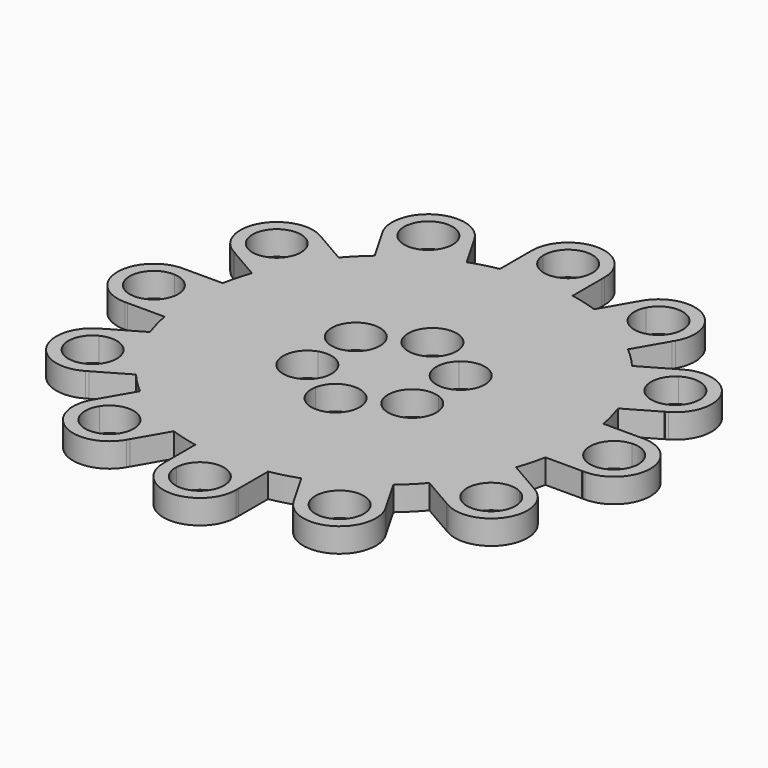
from build123d import *

# Parameters (mm, degrees)
F1_DEPTH = 1


with BuildPart() as f1:
    # F0 (on Top) → F1 (new body)
    with BuildSketch(Plane.XY):
        with BuildLine():
            ThreePointArc((9.4473684211, -0.9986139979), (8.5, 0), (9.4473684211, 0.9986139979))
            ThreePointArc((9.4473684211, 0.9986139979), (9.4177488558, 1.2473998912), (9.3815789474, 1.4953181783))
            ThreePointArc((9.3815789474, 1.4953181783), (9.3812055256, 1.4976591358), (9.3808315196, 1.5))
            Line((9.3808315196, 1.5), (7.8581168228, 1.5))
            ThreePointArc((7.8581168228, 1.5), (7.964450219, 0.7533476681), (8, 0))
            ThreePointArc((8, 0), (7.964450219, -0.7533476681), (7.8581168228, -1.5))
            Line((7.8581168228, -1.5), (9.3808315196, -1.5))
            ThreePointArc((9.3808315196, -1.5), (9.3812055256, -1.4976591358), (9.3815789474, -1.4953181783))
            ThreePointArc((9.3815789474, -1.4953181783), (9.4177488558, -1.2473998912), (9.4473684211, -0.9986139979))
        make_face()
        with BuildLine():
            ThreePointArc((9.3815789474, 1.4953181783), (9.4177488558, 1.2473998912), (9.4473684211, 0.9986139979))
            ThreePointArc((9.4473684211, 0.9986139979), (10.1882472016, 0.7254762501), (10.5, 0))
            ThreePointArc((10.5, 0), (10.1882472016, -0.7254762501), (9.4473684211, -0.9986139979))
            ThreePointArc((9.4473684211, -0.9986139979), (9.4177488558, -1.2473998912), (9.3815789474, -1.4953181783))
            ThreePointArc((9.3815789474, -1.4953181783), (9.4407432173, -1.4988290876), (9.5, -1.5))
            ThreePointArc((9.5, -1.5), (11, 0), (9.5, 1.5))
            ThreePointArc((9.5, 1.5), (9.4407432173, 1.4988290876), (9.3815789474, 1.4953181783))
        make_face()
        with BuildLine():
            Line((7.5553287944, 2.6300203057), (8.8740384046, 3.3913776541))
            ThreePointArc((8.8740384046, 3.3913776541), (8.8731918712, 3.393591905), (8.8723447852, 3.3958059446))
            ThreePointArc((8.8723447852, 3.3958059446), (8.7797097012, 3.6285944334), (8.6809680505, 3.8588591197))
            ThreePointArc((8.6809680505, 3.8588591197), (7.3612159322, 4.25), (7.6823540526, 5.5885093013))
            ThreePointArc((7.6823540526, 5.5885093013), (7.53230981, 5.7891544224), (7.3770266069, 5.9857730028))
            ThreePointArc((7.3770266069, 5.9857730028), (7.3755327354, 5.9876136206), (7.3740384046, 5.9894538655))
            Line((7.3740384046, 5.9894538655), (6.0553287944, 5.2280965171))
            ThreePointArc((6.0553287944, 5.2280965171), (6.9282032303, 4), (7.5553287944, 2.6300203057))
        make_face()
        with BuildLine():
            ThreePointArc((8, 0), (7.964450219, 0.7533476681), (7.8581168228, 1.5))
            ThreePointArc((7.8581168228, 1.5), (7.7274066103, 2.0705523608), (7.5553287944, 2.6300203057))
            ThreePointArc((7.5553287944, 2.6300203057), (6.9282032303, 4), (6.0553287944, 5.2280965171))
            ThreePointArc((6.0553287944, 5.2280965171), (5.6568542495, 5.6568542495), (5.2280965171, 6.0553287944))
            ThreePointArc((5.2280965171, 6.0553287944), (4, 6.9282032303), (2.6300203057, 7.5553287944))
            ThreePointArc((2.6300203057, 7.5553287944), (2.0705523608, 7.7274066103), (1.5, 7.8581168228))
            ThreePointArc((1.5, 7.8581168228), (0, 8), (-1.5, 7.8581168228))
            ThreePointArc((-1.5, 7.8581168228), (-2.0705523608, 7.7274066103), (-2.6300203057, 7.5553287944))
            ThreePointArc((-2.6300203057, 7.5553287944), (-4, 6.9282032303), (-5.2280965171, 6.0553287944))
            ThreePointArc((-5.2280965171, 6.0553287944), (-5.6568542495, 5.6568542495), (-6.0553287944, 5.2280965171))
            ThreePointArc((-6.0553287944, 5.2280965171), (-6.9282032303, 4), (-7.5553287944, 2.6300203057))
            ThreePointArc((-7.5553287944, 2.6300203057), (-7.7274066103, 2.0705523608), (-7.8581168228, 1.5))
            ThreePointArc((-7.8581168228, 1.5), (-8, 0), (-7.8581168228, -1.5))
            ThreePointArc((-7.8581168228, -1.5), (-7.7274066103, -2.0705523608), (-7.5553287944, -2.6300203057))
            ThreePointArc((-7.5553287944, -2.6300203057), (-6.9282032303, -4), (-6.0553287944, -5.2280965171))
            ThreePointArc((-6.0553287944, -5.2280965171), (-5.6568542495, -5.6568542495), (-5.2280965171, -6.0553287944))
            ThreePointArc((-5.2280965171, -6.0553287944), (-4, -6.9282032303), (-2.6300203057, -7.5553287944))
            ThreePointArc((-2.6300203057, -7.5553287944), (-2.0705523608, -7.7274066103), (-1.5, -7.8581168228))
            ThreePointArc((-1.5, -7.8581168228), (0, -8), (1.5, -7.8581168228))
            ThreePointArc((1.5, -7.8581168228), (2.0705523608, -7.7274066103), (2.6300203057, -7.5553287944))
            ThreePointArc((2.6300203057, -7.5553287944), (4, -6.9282032303), (5.2280965171, -6.0553287944))
            ThreePointArc((5.2280965171, -6.0553287944), (5.6568542495, -5.6568542495), (6.0553287944, -5.2280965171))
            ThreePointArc((6.0553287944, -5.2280965171), (6.9282032303, -4), (7.5553287944, -2.6300203057))
            ThreePointArc((7.5553287944, -2.6300203057), (7.7274066103, -2.0705523608), (7.8581168228, -1.5))
            ThreePointArc((7.8581168228, -1.5), (7.964450219, -0.7533476681), (8, 0))
        make_face()
        with BuildLine():
            ThreePointArc((2.4817563773, 0.3014718626), (2.4954349263, 0.1510116831), (2.5, 0))
            ThreePointArc((2.5, 0), (2.4954349263, -0.1510116831), (2.4817563773, -0.3014718626))
            ThreePointArc((2.4817563773, -0.3014718626), (2.9764490121, -0.6654886091), (3.1650635095, -1.25))
            ThreePointArc((3.1650635095, -1.25), (2.5754882716, -2.1618944646), (1.5019604801, -1.9985281374))
            ThreePointArc((1.5019604801, -1.9985281374), (1.25, -2.1650635095), (0.9797958971, -2.3))
            ThreePointArc((0.9797958971, -2.3), (0.994936153, -2.399491038), (1, -2.5))
            ThreePointArc((1, -2.5), (-0.100508962, -3.494936153), (-0.9797958971, -2.3))
            ThreePointArc((-0.9797958971, -2.3), (-1.25, -2.1650635095), (-1.5019604801, -1.9985281374))
            ThreePointArc((-1.5019604801, -1.9985281374), (-3.0310889132, -1.75), (-2.4817563773, -0.3014718626))
            ThreePointArc((-2.4817563773, -0.3014718626), (-2.5, 0), (-2.4817563773, 0.3014718626))
            ThreePointArc((-2.4817563773, 0.3014718626), (-3.0310889132, 1.75), (-1.5019604801, 1.9985281374))
            ThreePointArc((-1.5019604801, 1.9985281374), (-1.25, 2.1650635095), (-0.9797958971, 2.3))
            ThreePointArc((-0.9797958971, 2.3), (-0.100508962, 3.494936153), (1, 2.5))
            ThreePointArc((1, 2.5), (0.994936153, 2.399491038), (0.9797958971, 2.3))
            ThreePointArc((0.9797958971, 2.3), (1.25, 2.1650635095), (1.5019604801, 1.9985281374))
            ThreePointArc((1.5019604801, 1.9985281374), (2.5754882716, 2.1618944646), (3.1650635095, 1.25))
            ThreePointArc((3.1650635095, 1.25), (2.9764490121, 0.6654886091), (2.4817563773, 0.3014718626))
        make_face(mode=Mode.SUBTRACT)
        with BuildLine():
            ThreePointArc((8.8723447852, -3.3958059446), (8.8731918712, -3.393591905), (8.8740384046, -3.3913776541))
            Line((8.8740384046, -3.3913776541), (7.5553287944, -2.6300203057))
            ThreePointArc((7.5553287944, -2.6300203057), (6.9282032303, -4), (6.0553287944, -5.2280965171))
            Line((6.0553287944, -5.2280965171), (7.3740384046, -5.9894538655))
            ThreePointArc((7.3740384046, -5.9894538655), (7.3755327354, -5.9876136206), (7.3770266069, -5.9857730028))
            ThreePointArc((7.3770266069, -5.9857730028), (7.53230981, -5.7891544224), (7.6823540526, -5.5885093013))
            ThreePointArc((7.6823540526, -5.5885093013), (7.3612159322, -4.25), (8.6809680505, -3.8588591197))
            ThreePointArc((8.6809680505, -3.8588591197), (8.7797097012, -3.6285944334), (8.8723447852, -3.3958059446))
        make_face()
        with BuildLine():
            ThreePointArc((8.6809680505, 3.8588591197), (8.7797097012, 3.6285944334), (8.8723447852, 3.3958059446))
            ThreePointArc((8.8723447852, 3.3958059446), (8.9253380006, 3.4223475429), (8.977241336, 3.4509618943))
            ThreePointArc((8.977241336, 3.4509618943), (9.5262794416, 5.5), (7.477241336, 6.0490381057))
            ThreePointArc((7.477241336, 6.0490381057), (7.4265089131, 6.0183956744), (7.3770266069, 5.9857730028))
            ThreePointArc((7.3770266069, 5.9857730028), (7.53230981, 5.7891544224), (7.6823540526, 5.5885093013))
            ThreePointArc((7.6823540526, 5.5885093013), (8.7042700126, 5.6288877299), (9.227241336, 4.75))
            ThreePointArc((9.227241336, 4.75), (9.0798041532, 4.2273752372), (8.6809680505, 3.8588591197))
        make_face()
        with BuildLine():
            ThreePointArc((8.977241336, -3.4509618943), (8.9253380006, -3.4223475429), (8.8723447852, -3.3958059446))
            ThreePointArc((8.8723447852, -3.3958059446), (8.7797097012, -3.6285944334), (8.6809680505, -3.8588591197))
            ThreePointArc((8.6809680505, -3.8588591197), (9.0798041532, -4.2273752372), (9.227241336, -4.75))
            ThreePointArc((9.227241336, -4.75), (8.7042700126, -5.6288877299), (7.6823540526, -5.5885093013))
            ThreePointArc((7.6823540526, -5.5885093013), (7.53230981, -5.7891544224), (7.3770266069, -5.9857730028))
            ThreePointArc((7.3770266069, -5.9857730028), (7.4265089131, -6.0183956744), (7.477241336, -6.0490381057))
            ThreePointArc((7.477241336, -6.0490381057), (9.5262794416, -5.5), (8.977241336, -3.4509618943))
        make_face()
        with BuildLine():
            ThreePointArc((2.6300203057, 7.5553287944), (4, 6.9282032303), (5.2280965171, 6.0553287944))
            Line((5.2280965171, 6.0553287944), (5.9894538655, 7.3740384046))
            ThreePointArc((5.9894538655, 7.3740384046), (5.9876136206, 7.3755327354), (5.9857730028, 7.3770266069))
            ThreePointArc((5.9857730028, 7.3770266069), (5.7891544224, 7.53230981), (5.5885093013, 7.6823540526))
            ThreePointArc((5.5885093013, 7.6823540526), (4.25, 7.3612159322), (3.8588591197, 8.6809680505))
            ThreePointArc((3.8588591197, 8.6809680505), (3.6285944334, 8.7797097012), (3.3958059446, 8.8723447852))
            ThreePointArc((3.3958059446, 8.8723447852), (3.393591905, 8.8731918712), (3.3913776541, 8.8740384046))
            Line((3.3913776541, 8.8740384046), (2.6300203057, 7.5553287944))
        make_face()
        with BuildLine():
            Line((5.9894538655, -7.3740384046), (5.2280965171, -6.0553287944))
            ThreePointArc((5.2280965171, -6.0553287944), (4, -6.9282032303), (2.6300203057, -7.5553287944))
            Line((2.6300203057, -7.5553287944), (3.3913776541, -8.8740384046))
            ThreePointArc((3.3913776541, -8.8740384046), (3.393591905, -8.8731918712), (3.3958059446, -8.8723447852))
            ThreePointArc((3.3958059446, -8.8723447852), (3.6285944334, -8.7797097012), (3.8588591197, -8.6809680505))
            ThreePointArc((3.8588591197, -8.6809680505), (4.25, -7.3612159322), (5.5885093013, -7.6823540526))
            ThreePointArc((5.5885093013, -7.6823540526), (5.7891544224, -7.53230981), (5.9857730028, -7.3770266069))
            ThreePointArc((5.9857730028, -7.3770266069), (5.9876136206, -7.3755327354), (5.9894538655, -7.3740384046))
        make_face()
        with BuildLine():
            ThreePointArc((5.5885093013, 7.6823540526), (5.7891544224, 7.53230981), (5.9857730028, 7.3770266069))
            ThreePointArc((5.9857730028, 7.3770266069), (6.0183956744, 7.4265089131), (6.0490381057, 7.477241336))
            ThreePointArc((6.0490381057, 7.477241336), (5.5, 9.5262794416), (3.4509618943, 8.977241336))
            ThreePointArc((3.4509618943, 8.977241336), (3.4223475429, 8.9253380006), (3.3958059446, 8.8723447852))
            ThreePointArc((3.3958059446, 8.8723447852), (3.6285944334, 8.7797097012), (3.8588591197, 8.6809680505))
            ThreePointArc((3.8588591197, 8.6809680505), (4.9833014356, 9.1996457992), (5.75, 8.227241336))
            ThreePointArc((5.75, 8.227241336), (5.7087776857, 7.9430840743), (5.5885093013, 7.6823540526))
        make_face()
        with BuildLine():
            ThreePointArc((-1.5, 7.8581168228), (0, 8), (1.5, 7.8581168228))
            Line((1.5, 7.8581168228), (1.5, 9.3808315196))
            ThreePointArc((1.5, 9.3808315196), (1.4976591358, 9.3812055256), (1.4953181783, 9.3815789474))
            ThreePointArc((1.4953181783, 9.3815789474), (1.2473998912, 9.4177488558), (0.9986139979, 9.4473684211))
            ThreePointArc((0.9986139979, 9.4473684211), (0, 8.5), (-0.9986139979, 9.4473684211))
            ThreePointArc((-0.9986139979, 9.4473684211), (-1.2473998912, 9.4177488558), (-1.4953181783, 9.3815789474))
            ThreePointArc((-1.4953181783, 9.3815789474), (-1.4976591358, 9.3812055256), (-1.5, 9.3808315196))
            Line((-1.5, 9.3808315196), (-1.5, 7.8581168228))
        make_face()
        with BuildLine():
            ThreePointArc((6.0490381057, -7.477241336), (6.0183956744, -7.4265089131), (5.9857730028, -7.3770266069))
            ThreePointArc((5.9857730028, -7.3770266069), (5.7891544224, -7.53230981), (5.5885093013, -7.6823540526))
            ThreePointArc((5.5885093013, -7.6823540526), (5.7087776857, -7.9430840743), (5.75, -8.227241336))
            ThreePointArc((5.75, -8.227241336), (4.9833014356, -9.1996457992), (3.8588591197, -8.6809680505))
            ThreePointArc((3.8588591197, -8.6809680505), (3.6285944334, -8.7797097012), (3.3958059446, -8.8723447852))
            ThreePointArc((3.3958059446, -8.8723447852), (3.4223475429, -8.9253380006), (3.4509618943, -8.977241336))
            ThreePointArc((3.4509618943, -8.977241336), (5.5, -9.5262794416), (6.0490381057, -7.477241336))
        make_face()
        with BuildLine():
            Line((1.5, -9.3808315196), (1.5, -7.8581168228))
            ThreePointArc((1.5, -7.8581168228), (0, -8), (-1.5, -7.8581168228))
            Line((-1.5, -7.8581168228), (-1.5, -9.3808315196))
            ThreePointArc((-1.5, -9.3808315196), (-1.4976591358, -9.3812055256), (-1.4953181783, -9.3815789474))
            ThreePointArc((-1.4953181783, -9.3815789474), (-1.2473998912, -9.4177488558), (-0.9986139979, -9.4473684211))
            ThreePointArc((-0.9986139979, -9.4473684211), (0, -8.5), (0.9986139979, -9.4473684211))
            ThreePointArc((0.9986139979, -9.4473684211), (1.2473998912, -9.4177488558), (1.4953181783, -9.3815789474))
            ThreePointArc((1.4953181783, -9.3815789474), (1.4976591358, -9.3812055256), (1.5, -9.3808315196))
        make_face()
        with BuildLine():
            ThreePointArc((-5.2280965171, 6.0553287944), (-4, 6.9282032303), (-2.6300203057, 7.5553287944))
            Line((-2.6300203057, 7.5553287944), (-3.3913776541, 8.8740384046))
            ThreePointArc((-3.3913776541, 8.8740384046), (-3.393591905, 8.8731918712), (-3.3958059446, 8.8723447852))
            ThreePointArc((-3.3958059446, 8.8723447852), (-3.6285944334, 8.7797097012), (-3.8588591197, 8.6809680505))
            ThreePointArc((-3.8588591197, 8.6809680505), (-3.7775955368, 8.4605427716), (-3.75, 8.227241336))
            ThreePointArc((-3.75, 8.227241336), (-4.4658427384, 7.2684636502), (-5.5885093013, 7.6823540526))
            ThreePointArc((-5.5885093013, 7.6823540526), (-5.7910337944, 7.5308649963), (-5.9894538655, 7.3740384046))
            Line((-5.9894538655, 7.3740384046), (-5.2280965171, 6.0553287944))
        make_face()
        with BuildLine():
            ThreePointArc((0.9986139979, 9.4473684211), (1.2473998912, 9.4177488558), (1.4953181783, 9.3815789474))
            ThreePointArc((1.4953181783, 9.3815789474), (1.4988290876, 9.4407432173), (1.5, 9.5))
            ThreePointArc((1.5, 9.5), (0, 11), (-1.5, 9.5))
            ThreePointArc((-1.5, 9.5), (-1.4988290876, 9.4407432173), (-1.4953181783, 9.3815789474))
            ThreePointArc((-1.4953181783, 9.3815789474), (-1.2473998912, 9.4177488558), (-0.9986139979, 9.4473684211))
            ThreePointArc((-0.9986139979, 9.4473684211), (-0.0263249127, 10.4996534394), (1, 9.5))
            ThreePointArc((1, 9.5), (0.9996534394, 9.4736750873), (0.9986139979, 9.4473684211))
        make_face()
        with BuildLine():
            Line((-3.3913776541, -8.8740384046), (-2.6300203057, -7.5553287944))
            ThreePointArc((-2.6300203057, -7.5553287944), (-4, -6.9282032303), (-5.2280965171, -6.0553287944))
            Line((-5.2280965171, -6.0553287944), (-5.9894538655, -7.3740384046))
            ThreePointArc((-5.9894538655, -7.3740384046), (-5.9876136206, -7.3755327354), (-5.9857730028, -7.3770266069))
            ThreePointArc((-5.9857730028, -7.3770266069), (-5.7891544224, -7.53230981), (-5.5885093013, -7.6823540526))
            ThreePointArc((-5.5885093013, -7.6823540526), (-4.4658427384, -7.2684636502), (-3.75, -8.227241336))
            ThreePointArc((-3.75, -8.227241336), (-3.7775955368, -8.4605427716), (-3.8588591197, -8.6809680505))
            ThreePointArc((-3.8588591197, -8.6809680505), (-3.6285944334, -8.7797097012), (-3.3958059446, -8.8723447852))
            ThreePointArc((-3.3958059446, -8.8723447852), (-3.393591905, -8.8731918712), (-3.3913776541, -8.8740384046))
        make_face()
        with BuildLine():
            ThreePointArc((1.5, -9.5), (1.4988290876, -9.4407432173), (1.4953181783, -9.3815789474))
            ThreePointArc((1.4953181783, -9.3815789474), (1.2473998912, -9.4177488558), (0.9986139979, -9.4473684211))
            ThreePointArc((0.9986139979, -9.4473684211), (0.9996534394, -9.4736750873), (1, -9.5))
            ThreePointArc((1, -9.5), (-0.0263249127, -10.4996534394), (-0.9986139979, -9.4473684211))
            ThreePointArc((-0.9986139979, -9.4473684211), (-1.2473998912, -9.4177488558), (-1.4953181783, -9.3815789474))
            ThreePointArc((-1.4953181783, -9.3815789474), (-1.4988290876, -9.4407432173), (-1.5, -9.5))
            ThreePointArc((-1.5, -9.5), (0, -11), (1.5, -9.5))
        make_face()
        with BuildLine():
            ThreePointArc((-7.5553287944, 2.6300203057), (-6.9282032303, 4), (-6.0553287944, 5.2280965171))
            Line((-6.0553287944, 5.2280965171), (-7.3740384046, 5.9894538655))
            ThreePointArc((-7.3740384046, 5.9894538655), (-7.3755327354, 5.9876136206), (-7.3770266069, 5.9857730028))
            ThreePointArc((-7.3770266069, 5.9857730028), (-7.53230981, 5.7891544224), (-7.6823540526, 5.5885093013))
            ThreePointArc((-7.6823540526, 5.5885093013), (-7.3483536061, 5.2270286766), (-7.227241336, 4.75))
            ThreePointArc((-7.227241336, 4.75), (-7.7046165731, 3.8974371828), (-8.6809680505, 3.8588591197))
            ThreePointArc((-8.6809680505, 3.8588591197), (-8.7797097012, 3.6285944334), (-8.8723447852, 3.3958059446))
            ThreePointArc((-8.8723447852, 3.3958059446), (-8.8731918712, 3.393591905), (-8.8740384046, 3.3913776541))
            Line((-8.8740384046, 3.3913776541), (-7.5553287944, 2.6300203057))
        make_face()
        with BuildLine():
            Line((-6.0490381057, 7.477241336), (-5.9894538655, 7.3740384046))
            ThreePointArc((-5.9894538655, 7.3740384046), (-5.7910337944, 7.5308649963), (-5.5885093013, 7.6823540526))
            ThreePointArc((-5.5885093013, 7.6823540526), (-5.25, 9.0932667397), (-3.8588591197, 8.6809680505))
            ThreePointArc((-3.8588591197, 8.6809680505), (-3.6285944334, 8.7797097012), (-3.3958059446, 8.8723447852))
            ThreePointArc((-3.3958059446, 8.8723447852), (-3.4223475429, 8.9253380006), (-3.4509618943, 8.977241336))
            ThreePointArc((-3.4509618943, 8.977241336), (-5.5, 9.5262794416), (-6.0490381057, 7.477241336))
        make_face()
        with BuildLine():
            Line((-7.3740384046, -5.9894538655), (-6.0553287944, -5.2280965171))
            ThreePointArc((-6.0553287944, -5.2280965171), (-6.9282032303, -4), (-7.5553287944, -2.6300203057))
            Line((-7.5553287944, -2.6300203057), (-8.8740384046, -3.3913776541))
            ThreePointArc((-8.8740384046, -3.3913776541), (-8.8731918712, -3.393591905), (-8.8723447852, -3.3958059446))
            ThreePointArc((-8.8723447852, -3.3958059446), (-8.7797097012, -3.6285944334), (-8.6809680505, -3.8588591197))
            ThreePointArc((-8.6809680505, -3.8588591197), (-7.7046165731, -3.8974371828), (-7.227241336, -4.75))
            ThreePointArc((-7.227241336, -4.75), (-7.3483536061, -5.2270286766), (-7.6823540526, -5.5885093013))
            ThreePointArc((-7.6823540526, -5.5885093013), (-7.53230981, -5.7891544224), (-7.3770266069, -5.9857730028))
            ThreePointArc((-7.3770266069, -5.9857730028), (-7.3755327354, -5.9876136206), (-7.3740384046, -5.9894538655))
        make_face()
        with BuildLine():
            ThreePointArc((-3.4509618943, -8.977241336), (-3.4223475429, -8.9253380006), (-3.3958059446, -8.8723447852))
            ThreePointArc((-3.3958059446, -8.8723447852), (-3.6285944334, -8.7797097012), (-3.8588591197, -8.6809680505))
            ThreePointArc((-3.8588591197, -8.6809680505), (-5.25, -9.0932667397), (-5.5885093013, -7.6823540526))
            ThreePointArc((-5.5885093013, -7.6823540526), (-5.7891544224, -7.53230981), (-5.9857730028, -7.3770266069))
            ThreePointArc((-5.9857730028, -7.3770266069), (-6.0183956744, -7.4265089131), (-6.0490381057, -7.477241336))
            ThreePointArc((-6.0490381057, -7.477241336), (-5.5, -9.5262794416), (-3.4509618943, -8.977241336))
        make_face()
        with BuildLine():
            ThreePointArc((-7.8581168228, -1.5), (-8, 0), (-7.8581168228, 1.5))
            Line((-7.8581168228, 1.5), (-9.3808315196, 1.5))
            ThreePointArc((-9.3808315196, 1.5), (-9.3812055256, 1.4976591358), (-9.3815789474, 1.4953181783))
            ThreePointArc((-9.3815789474, 1.4953181783), (-9.4177488558, 1.2473998912), (-9.4473684211, 0.9986139979))
            ThreePointArc((-9.4473684211, 0.9986139979), (-8.7745237499, 0.6882472016), (-8.5, 0))
            ThreePointArc((-8.5, 0), (-8.7745237499, -0.6882472016), (-9.4473684211, -0.9986139979))
            ThreePointArc((-9.4473684211, -0.9986139979), (-9.4177488558, -1.2473998912), (-9.3815789474, -1.4953181783))
            ThreePointArc((-9.3815789474, -1.4953181783), (-9.3812055256, -1.4976591358), (-9.3808315196, -1.5))
            Line((-9.3808315196, -1.5), (-7.8581168228, -1.5))
        make_face()
        with BuildLine():
            ThreePointArc((-7.6823540526, 5.5885093013), (-7.53230981, 5.7891544224), (-7.3770266069, 5.9857730028))
            ThreePointArc((-7.3770266069, 5.9857730028), (-7.4265089131, 6.0183956744), (-7.477241336, 6.0490381057))
            ThreePointArc((-7.477241336, 6.0490381057), (-9.5262794416, 5.5), (-8.977241336, 3.4509618943))
            ThreePointArc((-8.977241336, 3.4509618943), (-8.9253380006, 3.4223475429), (-8.8723447852, 3.3958059446))
            ThreePointArc((-8.8723447852, 3.3958059446), (-8.7797097012, 3.6285944334), (-8.6809680505, 3.8588591197))
            ThreePointArc((-8.6809680505, 3.8588591197), (-9.0932667397, 5.25), (-7.6823540526, 5.5885093013))
        make_face()
        with BuildLine():
            ThreePointArc((-7.477241336, -6.0490381057), (-7.4265089131, -6.0183956744), (-7.3770266069, -5.9857730028))
            ThreePointArc((-7.3770266069, -5.9857730028), (-7.53230981, -5.7891544224), (-7.6823540526, -5.5885093013))
            ThreePointArc((-7.6823540526, -5.5885093013), (-9.0932667397, -5.25), (-8.6809680505, -3.8588591197))
            ThreePointArc((-8.6809680505, -3.8588591197), (-8.7797097012, -3.6285944334), (-8.8723447852, -3.3958059446))
            ThreePointArc((-8.8723447852, -3.3958059446), (-8.9253380006, -3.4223475429), (-8.977241336, -3.4509618943))
            ThreePointArc((-8.977241336, -3.4509618943), (-9.5262794416, -5.5), (-7.477241336, -6.0490381057))
        make_face()
        with BuildLine():
            ThreePointArc((-9.4473684211, 0.9986139979), (-9.4177488558, 1.2473998912), (-9.3815789474, 1.4953181783))
            ThreePointArc((-9.3815789474, 1.4953181783), (-9.4407432173, 1.4988290876), (-9.5, 1.5))
            ThreePointArc((-9.5, 1.5), (-11, 0), (-9.5, -1.5))
            ThreePointArc((-9.5, -1.5), (-9.4407432173, -1.4988290876), (-9.3815789474, -1.4953181783))
            ThreePointArc((-9.3815789474, -1.4953181783), (-9.4177488558, -1.2473998912), (-9.4473684211, -0.9986139979))
            ThreePointArc((-9.4473684211, -0.9986139979), (-10.5, 0), (-9.4473684211, 0.9986139979))
        make_face()
        with BuildLine():
            ThreePointArc((2.4817563773, -0.3014718626), (2.4954349263, -0.1510116831), (2.5, 0))
            ThreePointArc((2.5, 0), (2.4954349263, 0.1510116831), (2.4817563773, 0.3014718626))
            ThreePointArc((2.4817563773, 0.3014718626), (1.2990381057, 0.75), (1.5019604801, 1.9985281374))
            ThreePointArc((1.5019604801, 1.9985281374), (1.25, 2.1650635095), (0.9797958971, 2.3))
            ThreePointArc((0.9797958971, 2.3), (0, 1.5), (-0.9797958971, 2.3))
            ThreePointArc((-0.9797958971, 2.3), (-1.25, 2.1650635095), (-1.5019604801, 1.9985281374))
            ThreePointArc((-1.5019604801, 1.9985281374), (-1.2531690448, 1.6604247621), (-1.1650635095, 1.25))
            ThreePointArc((-1.1650635095, 1.25), (-1.5805521186, 0.4386144974), (-2.4817563773, 0.3014718626))
            ThreePointArc((-2.4817563773, 0.3014718626), (-2.5, 0), (-2.4817563773, -0.3014718626))
            ThreePointArc((-2.4817563773, -0.3014718626), (-1.5805521186, -0.4386144974), (-1.1650635095, -1.25))
            ThreePointArc((-1.1650635095, -1.25), (-1.2531690448, -1.6604247621), (-1.5019604801, -1.9985281374))
            ThreePointArc((-1.5019604801, -1.9985281374), (-1.25, -2.1650635095), (-0.9797958971, -2.3))
            ThreePointArc((-0.9797958971, -2.3), (0, -1.5), (0.9797958971, -2.3))
            ThreePointArc((0.9797958971, -2.3), (1.25, -2.1650635095), (1.5019604801, -1.9985281374))
            ThreePointArc((1.5019604801, -1.9985281374), (1.2990381057, -0.75), (2.4817563773, -0.3014718626))
        make_face()
    extrude(amount=F1_DEPTH)


solid = f1.part
